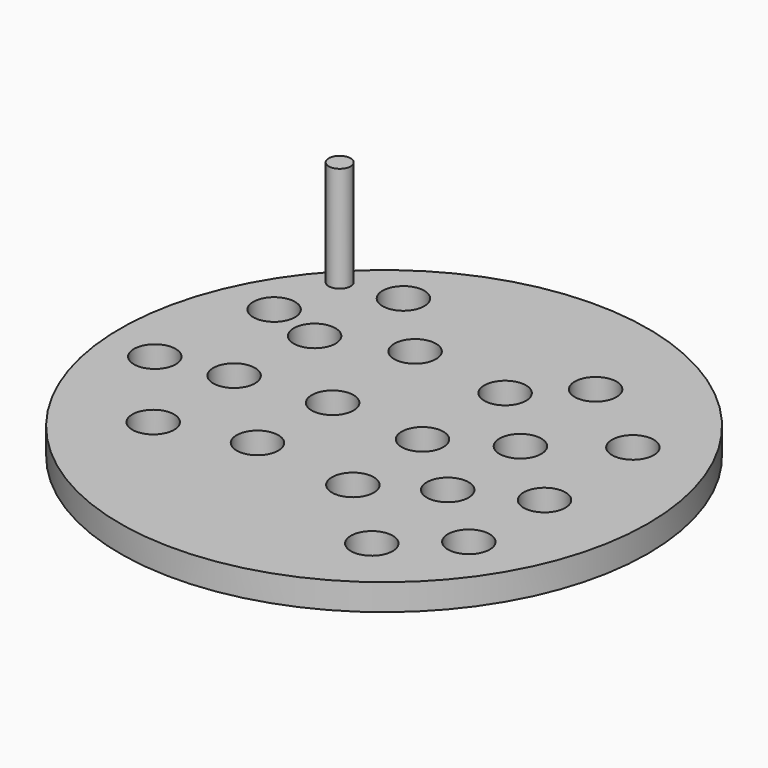
from build123d import *

# Parameters (mm, degrees)
F0_R     = 63.5
F1_DEPTH = 6.35
F2_R     = 5.0272245411
F3_DEPTH = 25.4
F4_R     = 2.641238627
F5_DEPTH = 25.4


# Not quite as in the source:
# - the program builds the solid bodies; features that only make, move or delete a surface that nothing else refers to are left out


with BuildPart() as f1:
    # F0 (on Top) → F1 (new body)
    with BuildSketch(Plane.XY):
        Circle(F0_R)
    extrude(amount=F1_DEPTH)

    # F2 (on face) → F3 (cut)
    with BuildSketch(Plane.XY.offset(6.35)):
        with Locations((-51.2941852212, -4.8283813521)):
            Circle(F2_R)
        with Locations((-45.7605943084, 24.1383034736)):
            Circle(F2_R)
        with Locations((-29.6111274511, 42.8337752819)):
            Circle(F2_R)
        with Locations((-33.1189669669, 20.5034371465)):
            Circle(F2_R)
        with Locations((-34.8243303597, -1.5672247391)):
            Circle(F2_R)
        with Locations((-34.8841510713, -25.8116889745)):
            Circle(F2_R)
        with Locations((-14.3142268062, -20.1833639294)):
            Circle(F2_R)
        with Locations((-13.4874591604, 1.3800424058)):
            Circle(F2_R)
        with Locations((-14.4421327859, 27.3816790432)):
            Circle(F2_R)
        with Locations((21.6737631708, 36.5187302232)):
            Circle(F2_R)
        with Locations((9.3525275588, 24.7192624956)):
            Circle(F2_R)
        with Locations((8.9998366311, 0.3057096619)):
            Circle(F2_R)
        with Locations((10.3590181097, -22.3385263234)):
            Circle(F2_R)
        with Locations((28.006831184, -38.7023799121)):
            Circle(F2_R)
        with Locations((25.5425348878, -12.7913486212)):
            Circle(F2_R)
        with Locations((25.1072477549, 9.6053304151)):
            Circle(F2_R)
        with Locations((41.9120192528, 22.4314276129)):
            Circle(F2_R)
        with Locations((42.3262864351, -4.6631796286)):
            Circle(F2_R)
        with Locations((41.8376736343, -26.8122982234)):
            Circle(F2_R)
    extrude(amount=-F3_DEPTH, mode=Mode.SUBTRACT)

    # F4 (on face) → F5 (join)
    with BuildSketch(Plane.XY.offset(6.35)):
        with Locations((-43.0771894753, 40.4972620308)):
            Circle(F4_R)
    extrude(amount=F5_DEPTH)


solid = f1.part
